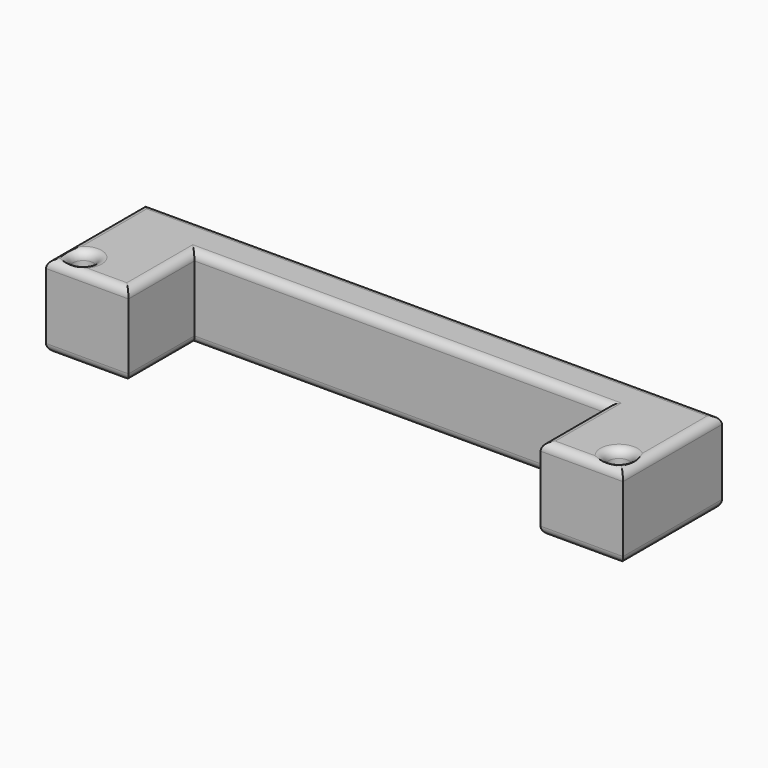
from build123d import *

# Parameters (mm, degrees)
F1_DEPTH     = 20
F3_D         = 5
F5_T1_DEPTH  = 150
F5_T3_DEPTH  = 40
F5_T5_DEPTH  = 25
F5_T7_DEPTH  = 100
F5_T9_DEPTH  = 30
F5_T11_DEPTH = 30
F5_T25_DEPTH = 30
F5_T29_DEPTH = 105
F5_T36_DEPTH = 105
F5_T40_DEPTH = 30
F5_T47_DEPTH = 30
F5_T51_DEPTH = 105
F5_T58_DEPTH = 105
F5_T62_DEPTH = 30


# Not quite as in the source:
# - a fillet or chamfer that OpenCascade refuses, or shapes differently, is made with other operations: its cross-section is extruded or revolved along the edge and cut away or added


with BuildPart() as f1:
    # F0 (on Top) → F1 (new body)
    with BuildSketch(Plane.XY):
        Polygon((70, 30), (0, 30), (0, 20), (50, 20), (50, 0), (70, 0), align=None)
    extrude(amount=F1_DEPTH)

    # F3 (through all)
    with Locations(Plane(origin=(0, 0, 0), x_dir=(1, 0, 0), z_dir=(0, 0, -1))):
        with Locations((65, -5)):
            Hole(F3_D / 2)

    # F4: F1 across face


with BuildPart() as f1_1:
    add(f1.part)
    add(f1.part.mirror(Plane(origin=(0, 25, 10), x_dir=(0, -1, 0), z_dir=(-1, 0, 0))))

    # F5: fillet of radius 2 on 20 edges, made by hand

    # F5_s2 → F5_t1 (cut)
    with BuildSketch(Plane.YZ.offset(-75)):
        with BuildLine():
            ThreePointArc((30, 18), (29.4142135624, 19.4142135624), (28, 20))
            Line((28, 20), (30, 20))
            Line((30, 20), (30, 18))
        make_face()
        with BuildLine():
            ThreePointArc((30, 2), (29.4142135624, 0.5857864376), (28, 0))
            Line((28, 0), (30, 0))
            Line((30, 0), (30, 2))
        make_face()
    extrude(amount=F5_T1_DEPTH, mode=Mode.SUBTRACT)

    # F5_s4 → F5_t3 (cut)
    with BuildSketch(Plane.XZ.offset(-35)):
        with BuildLine():
            ThreePointArc((68, 20), (69.4142135624, 19.4142135624), (70, 18))
            Line((70, 18), (70, 20))
            Line((70, 20), (68, 20))
        make_face()
        with BuildLine():
            ThreePointArc((-70, 18), (-69.4142135624, 19.4142135624), (-68, 20))
            Line((-68, 20), (-70, 20))
            Line((-70, 20), (-70, 18))
        make_face()
        with BuildLine():
            ThreePointArc((-68, 0), (-69.4142135624, 0.5857864376), (-70, 2))
            Line((-70, 2), (-70, 0))
            Line((-70, 0), (-68, 0))
        make_face()
        with BuildLine():
            ThreePointArc((68, 0), (69.4142135624, 0.5857864376), (70, 2))
            Line((70, 2), (70, 0))
            Line((70, 0), (68, 0))
        make_face()
    extrude(amount=F5_T3_DEPTH, mode=Mode.SUBTRACT)

    # F5_s6 → F5_t5 (cut)
    with BuildSketch(Plane.XZ.offset(-20)):
        with BuildLine():
            ThreePointArc((50, 18), (50.5857864376, 19.4142135624), (52, 20))
            Line((52, 20), (50, 20))
            Line((50, 20), (50, 18))
        make_face()
        with BuildLine():
            ThreePointArc((-50, 18), (-50.5857864376, 19.4142135624), (-52, 20))
            Line((-52, 20), (-50, 20))
            Line((-50, 20), (-50, 18))
        make_face()
        with BuildLine():
            ThreePointArc((-52, 0), (-50.5857864376, 0.5857864376), (-50, 2))
            Line((-50, 2), (-50, 0))
            Line((-50, 0), (-52, 0))
        make_face()
        with BuildLine():
            ThreePointArc((52, 0), (50.5857864376, 0.5857864376), (50, 2))
            Line((50, 2), (50, 0))
            Line((50, 0), (52, 0))
        make_face()
    extrude(amount=F5_T5_DEPTH, mode=Mode.SUBTRACT)

    # F5_s8 → F5_t7 (cut)
    with BuildSketch(Plane.YZ.offset(-50)):
        with BuildLine():
            ThreePointArc((20, 18), (20.5857864376, 19.4142135624), (22, 20))
            Line((22, 20), (20, 20))
            Line((20, 20), (20, 18))
        make_face()
        with BuildLine():
            ThreePointArc((22, 0), (20.5857864376, 0.5857864376), (20, 2))
            Line((20, 2), (20, 0))
            Line((20, 0), (22, 0))
        make_face()
    extrude(amount=F5_T7_DEPTH, mode=Mode.SUBTRACT)

    # F5_s10 → F5_t9 (cut)
    with BuildSketch(Plane.YZ.offset(-75)):
        with BuildLine():
            ThreePointArc((0, 18), (0.5857864376, 19.4142135624), (2, 20))
            Line((2, 20), (0, 20))
            Line((0, 20), (0, 18))
        make_face()
        with BuildLine():
            ThreePointArc((2, 0), (0.5857864376, 0.5857864376), (0, 2))
            Line((0, 2), (0, 0))
            Line((0, 0), (2, 0))
        make_face()
    extrude(amount=F5_T9_DEPTH, mode=Mode.SUBTRACT)

    # F5_s12 → F5_t11 (cut)
    with BuildSketch(Plane.YZ.offset(45)):
        with BuildLine():
            ThreePointArc((2, 0), (0.5857864376, 0.5857864376), (0, 2))
            Line((0, 2), (0, 0))
            Line((0, 0), (2, 0))
        make_face()
        with BuildLine():
            ThreePointArc((0, 18), (0.5857864376, 19.4142135624), (2, 20))
            Line((2, 20), (0, 20))
            Line((0, 20), (0, 18))
        make_face()
    extrude(amount=F5_T11_DEPTH, mode=Mode.SUBTRACT)

    # F5_s13 → F5_t14 (revolve, cut)
    with BuildSketch(Plane.XZ.offset(-5)):
        with BuildLine():
            ThreePointArc((69.5, 0), (68.0857864376, 0.5857864376), (67.5, 2))
            Line((67.5, 2), (67.5, 0))
            Line((67.5, 0), (69.5, 0))
        make_face()
    revolve(axis=Axis((65, 5, 0), (0, 0, -1)), mode=Mode.SUBTRACT)

    # F5_s15 → F5_t16 (revolve, cut)
    with BuildSketch(Plane.XZ.offset(-5)):
        with BuildLine():
            ThreePointArc((-69.5, 0), (-68.0857864376, 0.5857864376), (-67.5, 2))
            Line((-67.5, 2), (-67.5, 0))
            Line((-67.5, 0), (-69.5, 0))
        make_face()
    revolve(axis=Axis((-65, 5, 0), (0, 0, 1)), mode=Mode.SUBTRACT)

    # F5_s17 → F5_t18 (revolve, cut)
    with BuildSketch(Plane.XZ.offset(-5)):
        with BuildLine():
            ThreePointArc((67.5, 18), (68.0857864376, 19.4142135624), (69.5, 20))
            Line((69.5, 20), (67.5, 20))
            Line((67.5, 20), (67.5, 18))
        make_face()
    revolve(axis=Axis((65, 5, 20), (0, 0, -1)), mode=Mode.SUBTRACT)

    # F5_s19 → F5_t20 (revolve, cut)
    with BuildSketch(Plane.XZ.offset(-5)):
        with BuildLine():
            ThreePointArc((-67.5, 18), (-68.0857864376, 19.4142135624), (-69.5, 20))
            Line((-69.5, 20), (-67.5, 20))
            Line((-67.5, 20), (-67.5, 18))
        make_face()
    revolve(axis=Axis((-65, 5, 20), (0, 0, 1)), mode=Mode.SUBTRACT)


with BuildPart() as f5_tool23:
    # F5_s24 → F5_t25 (new body)
    with BuildSketch(Plane.XZ.offset(-25)):
        with BuildLine():
            ThreePointArc((50, 18), (50.5857864376, 19.4142135624), (52, 20))
            Line((52, 20), (50, 20))
            Line((50, 20), (50, 18))
        make_face()
    extrude(amount=F5_T25_DEPTH)

    split(bisect_by=Plane.XZ.offset(-20), keep=Keep.BOTTOM)


with BuildPart() as f5_tool27:
    # F5_s28 → F5_t29 (new body)
    with BuildSketch(Plane.YZ.offset(-50)):
        with BuildLine():
            ThreePointArc((20, 18), (20.5857864376, 19.4142135624), (22, 20))
            Line((22, 20), (20, 20))
            Line((20, 20), (20, 18))
        make_face()
    extrude(amount=F5_T29_DEPTH)

    split(bisect_by=Plane.YZ.offset(50), keep=Keep.TOP)


with BuildPart() as f5_tool23_1:
    add(f5_tool23.part)

    # F5_t31: intersect F5_tool27
    add(f5_tool27.part, mode=Mode.INTERSECT)


with BuildPart() as f1_2:
    add(f1_1.part)

    # F5_t21: cut F5_tool23
    add(f5_tool23_1.part, mode=Mode.SUBTRACT)


with BuildPart() as f5_tool34:
    # F5_s35 → F5_t36 (new body)
    with BuildSketch(Plane.YZ.offset(-55)):
        with BuildLine():
            ThreePointArc((20, 18), (20.5857864376, 19.4142135624), (22, 20))
            Line((22, 20), (20, 20))
            Line((20, 20), (20, 18))
        make_face()
    extrude(amount=F5_T36_DEPTH)

    split(bisect_by=Plane.YZ.offset(-50), keep=Keep.BOTTOM)


with BuildPart() as f5_tool38:
    # F5_s39 → F5_t40 (new body)
    with BuildSketch(Plane.XZ.offset(-25)):
        with BuildLine():
            ThreePointArc((-50, 18), (-50.5857864376, 19.4142135624), (-52, 20))
            Line((-52, 20), (-50, 20))
            Line((-50, 20), (-50, 18))
        make_face()
    extrude(amount=F5_T40_DEPTH)

    split(bisect_by=Plane.XZ.offset(-20), keep=Keep.BOTTOM)


with BuildPart() as f5_tool34_1:
    add(f5_tool34.part)

    # F5_t42: intersect F5_tool38
    add(f5_tool38.part, mode=Mode.INTERSECT)


with BuildPart() as f1_3:
    add(f1_2.part)

    # F5_t32: cut F5_tool34
    add(f5_tool34_1.part, mode=Mode.SUBTRACT)


with BuildPart() as f5_tool45:
    # F5_s46 → F5_t47 (new body)
    with BuildSketch(Plane.XZ.offset(-25)):
        with BuildLine():
            ThreePointArc((-52, 0), (-50.5857864376, 0.5857864376), (-50, 2))
            Line((-50, 2), (-50, 0))
            Line((-50, 0), (-52, 0))
        make_face()
    extrude(amount=F5_T47_DEPTH)

    split(bisect_by=Plane.XZ.offset(-20), keep=Keep.BOTTOM)


with BuildPart() as f5_tool49:
    # F5_s50 → F5_t51 (new body)
    with BuildSketch(Plane.YZ.offset(50)):
        with BuildLine():
            ThreePointArc((22, 0), (20.5857864376, 0.5857864376), (20, 2))
            Line((20, 2), (20, 0))
            Line((20, 0), (22, 0))
        make_face()
    extrude(amount=-F5_T51_DEPTH)

    split(bisect_by=Plane.YZ.offset(-50), keep=Keep.BOTTOM)


with BuildPart() as f5_tool45_1:
    add(f5_tool45.part)

    # F5_t53: intersect F5_tool49
    add(f5_tool49.part, mode=Mode.INTERSECT)


with BuildPart() as f1_4:
    add(f1_3.part)

    # F5_t43: cut F5_tool45
    add(f5_tool45_1.part, mode=Mode.SUBTRACT)


with BuildPart() as f5_tool56:
    # F5_s57 → F5_t58 (new body)
    with BuildSketch(Plane.YZ.offset(55)):
        with BuildLine():
            ThreePointArc((22, 0), (20.5857864376, 0.5857864376), (20, 2))
            Line((20, 2), (20, 0))
            Line((20, 0), (22, 0))
        make_face()
    extrude(amount=-F5_T58_DEPTH)

    split(bisect_by=Plane.YZ.offset(50), keep=Keep.TOP)


with BuildPart() as f5_tool60:
    # F5_s61 → F5_t62 (new body)
    with BuildSketch(Plane.XZ.offset(-25)):
        with BuildLine():
            ThreePointArc((52, 0), (50.5857864376, 0.5857864376), (50, 2))
            Line((50, 2), (50, 0))
            Line((50, 0), (52, 0))
        make_face()
    extrude(amount=F5_T62_DEPTH)

    split(bisect_by=Plane.XZ.offset(-20), keep=Keep.BOTTOM)


with BuildPart() as f5_tool56_1:
    add(f5_tool56.part)

    # F5_t64: intersect F5_tool60
    add(f5_tool60.part, mode=Mode.INTERSECT)


with BuildPart() as f1_5:
    add(f1_4.part)

    # F5_t54: cut F5_tool56
    add(f5_tool56_1.part, mode=Mode.SUBTRACT)


solid = f1_5.part
